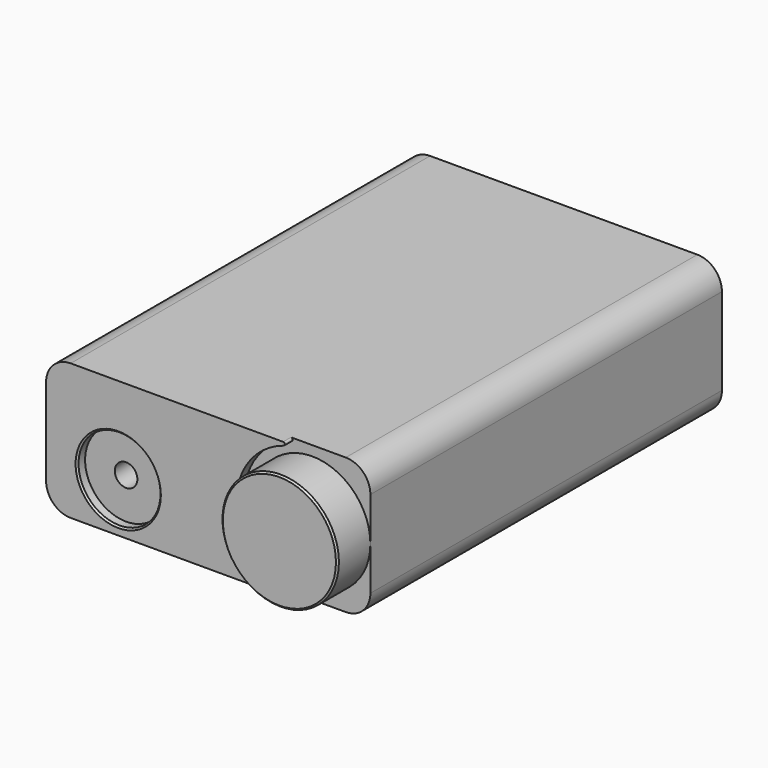
from build123d import *

# Parameters (mm, degrees)
F0_R     = 6.35
F0_R_2   = 9.017
F0_R_3   = 1.75
F1_DEPTH = 68.072
F2_DEPTH = 6.35
F3_DEPTH = 1.524
F4_DEPTH = 12.7
F5_R     = 0.2539
F6_SIZE  = 0.254
F7_R     = 3.81
F8_DEPTH = 2.286
F9_R     = 1.905


# Not quite as in the source:
# - a fillet or chamfer is up to 0.001 mm smaller than in the source, because OpenCascade refuses the exact size


with BuildPart() as f1:
    # F0 (on Front) → F1 (new body)
    with BuildSketch(Plane.XZ):
        with BuildLine():
            Line((-20.701, -10.541), (15.494, -10.541))
            ThreePointArc((15.494, -10.541), (4.953, 0), (15.494, 10.541))
            Line((15.494, 10.541), (-20.701, 10.541))
            ThreePointArc((-20.701, 10.541), (-23.3950768363, 9.4250768363), (-24.511, 6.731))
            Line((-24.511, 6.731), (-24.511, -6.731))
            ThreePointArc((-24.511, -6.731), (-23.3950768363, -9.4250768363), (-20.701, -10.541))
        make_face()
        with Locations((-13.335, -2.921)):
            Circle(F0_R, mode=Mode.SUBTRACT)
        with BuildLine():
            Line((15.494, -10.541), (20.701, -10.541))
            ThreePointArc((20.701, -10.541), (23.3950768363, -9.4250768363), (24.511, -6.731))
            Line((24.511, -6.731), (24.511, 0))
            Line((24.511, 0), (24.511, 6.731))
            ThreePointArc((24.511, 6.731), (23.3950768363, 9.4250768363), (20.701, 10.541))
            Line((20.701, 10.541), (15.494, 10.541))
            ThreePointArc((15.494, 10.541), (4.953, 0), (15.494, -10.541))
        make_face()
        with Locations((15.494, 0)):
            Circle(F0_R_2, mode=Mode.SUBTRACT)
        with Locations((15.494, 0)):
            Circle(F0_R_2)
        with Locations((-13.335, -2.921)):
            Circle(F0_R)
        with Locations((-13.335, -2.921)):
            Circle(F0_R_3, mode=Mode.SUBTRACT)
        with Locations((-13.335, -2.921)):
            Circle(F0_R_3)
    extrude(amount=-F1_DEPTH)

    # F0 (on Front) → F2 (join)
    with BuildSketch(Plane.XZ):
        with Locations((15.494, 0)):
            Circle(F0_R_2)
    extrude(amount=F2_DEPTH)

    # F0 (on Front) → F3 (join)
    with BuildSketch(Plane.XZ):
        with BuildLine():
            Line((-20.701, -10.541), (15.494, -10.541))
            ThreePointArc((15.494, -10.541), (4.953, 0), (15.494, 10.541))
            Line((15.494, 10.541), (-20.701, 10.541))
            ThreePointArc((-20.701, 10.541), (-23.3950768363, 9.4250768363), (-24.511, 6.731))
            Line((-24.511, 6.731), (-24.511, -6.731))
            ThreePointArc((-24.511, -6.731), (-23.3950768363, -9.4250768363), (-20.701, -10.541))
        make_face()
        with Locations((-13.335, -2.921)):
            Circle(F0_R, mode=Mode.SUBTRACT)
    extrude(amount=F3_DEPTH)

    # F0 (on Front) → F4 (cut)
    with BuildSketch(Plane.XZ):
        with Locations((-13.335, -2.921)):
            Circle(F0_R_3)
    extrude(amount=-F4_DEPTH, mode=Mode.SUBTRACT)

    # F5 (radius 0.254 in the source; OpenCascade refuses exactly that, so slightly less here)
    f5_edges = [f1.edges().sort_by_distance(p)[0] for p in [
        (15.494, -0.762, 10.541),
        (15.494, -0.762, -10.541),
    ]]
    fillet(f5_edges, radius=F5_R)

    # F6
    f6_edges = [f1.edges().sort_by_distance(p)[0] for p in [
        (6.477, -6.35, 0),
        (-19.685, -1.524, -2.921),
    ]]
    chamfer(f6_edges, length=F6_SIZE)

    # F7 (on face) → F8 (join)
    with BuildSketch(Plane(origin=(0, 0, -10.541), x_dir=(1, 0, 0), z_dir=(0, 0, -1))):
        with Locations((-14.605, -7.366)):
            Circle(F7_R)
        with Locations((14.605, -7.366)):
            Circle(F7_R)
        with Locations((-14.605, -60.706)):
            Circle(F7_R)
        with Locations((14.605, -59.182)):
            Circle(F7_R)
    extrude(amount=F8_DEPTH)

    # F9
    f9_edges = [f1.edges().sort_by_distance(p)[0] for p in [
        (-18.415, 7.366, -12.827),
        (10.795, 7.366, -12.827),
        (10.795, 59.182, -12.827),
        (-18.415, 60.706, -12.827),
    ]]
    fillet(f9_edges, radius=F9_R)


solid = f1.part
